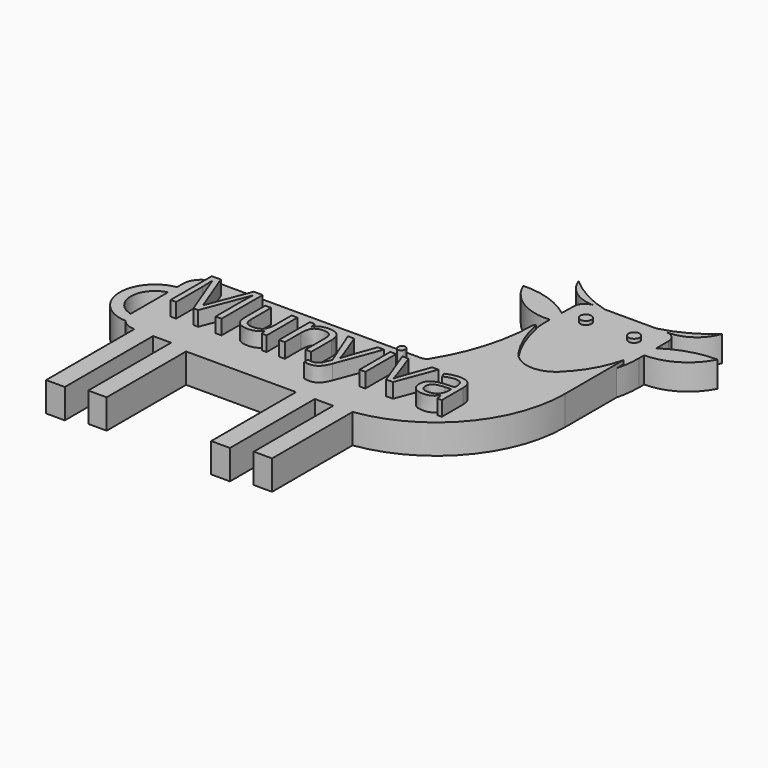
from build123d import *

# Parameters (mm, degrees)
F1_DEPTH     = 8
F3_DEPTH     = 7
F5_R         = 1.5
F6_DEPTH     = 1
F4_TEXT_SIZE = 19.5858165777
F7_DEPTH     = 4


# Not quite as in the source:
# - Text() gives the source's letters only with a copy of the font that has no kerning and outlines rounded to 1/6400 em; it was checked with that copy


with BuildPart() as f1:
    # F0 (on Top) → F1 (new body)
    with BuildSketch(Plane.XY):
        with BuildLine():
            Line((-45, 3.8386569105), (-45, 6.8960478014))
            ThreePointArc((-45, 6.8960478014), (-52.9829086733, -3.0701346322), (-43.8654525222, -12.0101355559))
            ThreePointArc((-43.8654525222, -12.0101355559), (-44.707826601, -10.5228091288), (-45, -8.8386569105))
            ThreePointArc((-45, -8.8386569105), (-50, -2.5), (-45, 3.8386569105))
        make_face()
        with BuildLine():
            Line((15.8297046912, 13.8386569105), (-40, 13.8386569105))
            ThreePointArc((-40, 13.8386569105), (-43.5355339059, 12.3741908164), (-45, 8.8386569105))
            Line((-45, 8.8386569105), (-45, 6.8960478014))
            Line((-45, 6.8960478014), (-45, 3.8386569105))
            Line((-45, 3.8386569105), (-45, 3.7625763263))
            Line((-45, 3.7625763263), (-45, -8.8386569105))
            ThreePointArc((-45, -8.8386569105), (-44.707826601, -10.5228091288), (-43.8654525222, -12.0101355559))
            ThreePointArc((-43.8654525222, -12.0101355559), (-42.1380606601, -13.3584684788), (-40, -13.8386569105))
            Line((-40, -13.8386569105), (-40, -41.7386569105))
            Line((-40, -41.7386569105), (-40, -43.8386569105))
            Line((-40, -43.8386569105), (-34.9, -43.8386569105))
            Line((-34.9, -43.8386569105), (-34.9, -41.7386569105))
            Line((-34.9, -41.7386569105), (-34.9, -13.8386569105))
            Line((-34.9, -13.8386569105), (-30, -13.8386569105))
            Line((-30, -13.8386569105), (-30, -40))
            Line((-30, -40), (-30, -42))
            Line((-30, -42), (-25, -42))
            Line((-25, -42), (-25, -40))
            Line((-25, -40), (-25, -15))
            Line((-25, -15), (4.9, -15))
            Line((4.9, -15), (4.9, -41.7386569105))
            Line((4.9, -41.7386569105), (4.9, -43.8386569105))
            Line((4.9, -43.8386569105), (10, -43.8386569105))
            Line((10, -43.8386569105), (10, -42.9))
            Line((10, -42.9), (10, -15))
            Line((10, -15), (15, -15))
            Line((15, -15), (15, -40))
            Line((15, -40), (15, -42))
            Line((15, -42), (19.9872285871, -42))
            Line((19.9872285871, -42), (19.9872285871, -40))
            Line((19.9872285871, -40), (19.9872285871, -14.6428571429))
            ThreePointArc((19.9872285871, -14.6428571429), (41.4532890256, -2.9177551197), (50, 20))
            Line((50, 20), (50, 39.8706895756))
            ThreePointArc((50, 39.8706895756), (47.2671677226, 33.027054972), (42.72400507, 27.2250398086))
            ThreePointArc((42.72400507, 27.2250398086), (36.352621039, 25.0437121367), (30.5730579932, 28.5004990673))
            ThreePointArc((30.5730579932, 28.5004990673), (27.3672069836, 34.4409303152), (25.4371913564, 40.9094111094))
            ThreePointArc((25.4371913564, 40.9094111094), (25.1136791278, 40.5576050767), (24.9903873882, 40.0958402083))
            ThreePointArc((24.9903873882, 40.0958402083), (22.960215899, 26.9405438101), (17.5309423867, 14.7870912665))
            ThreePointArc((17.5309423867, 14.7870912665), (16.8035806361, 14.0917838058), (15.8297046912, 13.8386569105))
        make_face()
    extrude(amount=F1_DEPTH)

    # F2 (on Top) → F3 (join)
    with BuildSketch(Plane.XY):
        with BuildLine():
            ThreePointArc((10.8507772448, 54.8047575814), (16.50976187, 48.1817938697), (24.9897626411, 46.1874663547))
            ThreePointArc((24.9897626411, 46.1874663547), (26.2936888702, 35.9615777639), (30.6891964287, 26.6369579654))
            ThreePointArc((30.6891964287, 26.6369579654), (36.4687594745, 23.1801710348), (42.8401435056, 25.3614987067))
            ThreePointArc((42.8401435056, 25.3614987067), (48.7619480085, 33.9274573056), (50.8473983026, 44.1301193289))
            Line((50.8473983026, 44.1301193289), (50.8473983026, 45.8717922632))
            ThreePointArc((50.8473983026, 45.8717922632), (58.711139834, 48.0958310645), (64.2452004325, 54.1090625381))
            ThreePointArc((64.2452004325, 54.1090625381), (57.2369150268, 53.0561633678), (50.8473983026, 49.9904274007))
            Line((50.8473983026, 49.9904274007), (50.8473983026, 54.1364588981))
            ThreePointArc((50.8473983026, 54.1364588981), (50.0250135915, 56.1999490613), (48.0087372004, 57.1321173834))
            ThreePointArc((48.0087372004, 57.1321173834), (53.911136747, 58.9236843212), (57.6394404208, 63.8377238221))
            ThreePointArc((57.6394404208, 63.8377238221), (51.7888401615, 59.7372514611), (45.1345727321, 57.1364588981))
            Line((45.1345727321, 57.1364588981), (31.171016995, 57.1364588981))
            ThreePointArc((31.171016995, 57.1364588981), (24.5167495656, 59.7372514611), (18.6661493063, 63.8377238221))
            ThreePointArc((18.6661493063, 63.8377238221), (22.2832798737, 59.0068055525), (28.0212728633, 57.1368212424))
            ThreePointArc((28.0212728633, 57.1368212424), (25.9466414457, 56.2186971047), (25.1080159398, 54.1106755888))
            Line((25.1080159398, 54.1106755888), (25.0488892904, 50.1490709718))
            ThreePointArc((25.0488892904, 50.1490709718), (18.3571930475, 53.7192100502), (10.8507772448, 54.8047575814))
        make_face()
        with BuildLine():
            ThreePointArc((47.8473983026, 57.1364588981), (47.928096953, 57.135373323), (48.0087372004, 57.1321173834))
            ThreePointArc((48.0087372004, 57.1321173834), (47.9280589925, 57.1339626397), (47.8473983026, 57.1364588981))
        make_face(mode=Mode.SUBTRACT)
        with BuildLine():
            ThreePointArc((47.8473983026, 57.1364588981), (47.9280589925, 57.1339626397), (48.0087372004, 57.1321173834))
            ThreePointArc((48.0087372004, 57.1321173834), (47.928096953, 57.135373323), (47.8473983026, 57.1364588981))
        make_face()
    extrude(amount=F3_DEPTH)

    # F5 (on face) → F6 (join)
    with BuildSketch(Plane.XY.offset(7)):
        with Locations((31.5901308308, 50.1490709718)):
            Circle(F5_R)
        with Locations((44.7154588963, 50.1490709718)):
            Circle(F5_R)
    extrude(amount=F6_DEPTH)

    # F4 (on face) → F7 (join)
    with BuildSketch(Plane.XY.offset(8)):
        with Locations((-39.4899267703, -4.5409915037)):
            Text('Munyiva', F4_TEXT_SIZE, font='Open Sans', text_align=(TextAlign.LEFT, TextAlign.BOTTOM))
    extrude(amount=F7_DEPTH)


solid = f1.part
